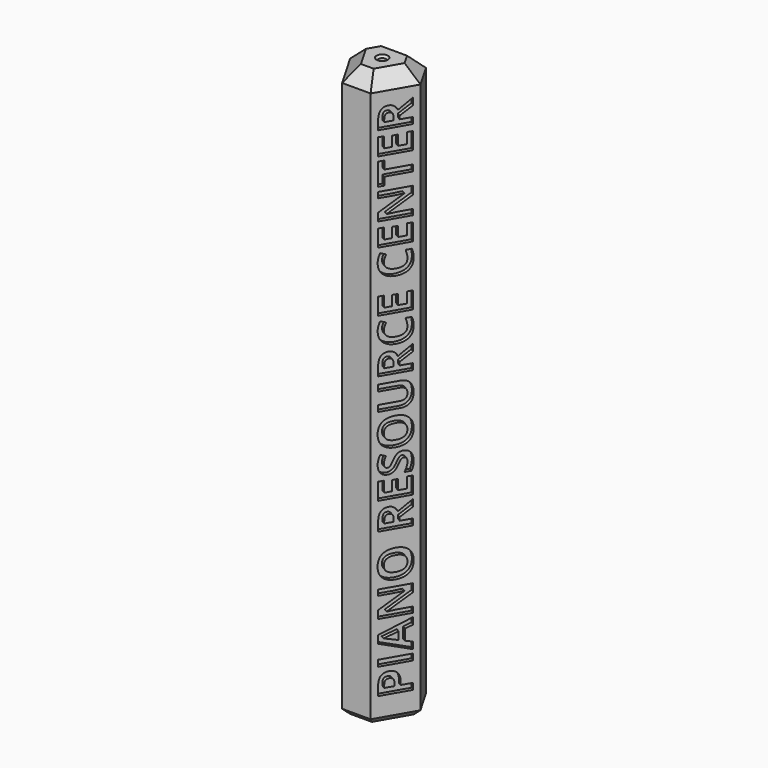
from build123d import *

# Parameters (mm, degrees)
F1_DEPTH        = 63.5
F3_D            = 4.064
F3_DEPTH        = 60.325
F3_CSINK_D      = 4.191
F3_CSINK_ANGLE  = 90
F3_TIP          = 1.2209487779
F4_SIZE         = 3.175
F5_TEXT_SIZE    = 4.5809615059
F6_DEPTH        = 0.4318
F7_TEXT_SIZE    = 4.5809615059
F8_DEPTH        = 0.4318
F9_TEXT_SIZE    = 4.5809615059
F10_DEPTH       = 0.4318
F12_D           = 0.79375
F12_CSINK_D     = 1.27
F12_CSINK_ANGLE = 90
F13_SIZE        = 0.635
F14_SIZE        = 1.524


# Not quite as in the source:
# - a feature names something its author has since deleted; it is built from what else it names
# - Text() gives the source's letters only with a copy of the font that has no kerning and outlines rounded to 1/6400 em; it was checked with that copy


with BuildPart() as f1:
    # F0 (on Top) → F1 (new body)
    with BuildSketch(Plane.XY):
        Polygon((-5.499261314, 3.175), (0, -6.35), (5.499261314, 3.175), align=None)
    extrude(amount=-F1_DEPTH)

    # F3
    with Locations(Plane(origin=(0, 0, -63.5), x_dir=(1, 0, 0), z_dir=(0, 0, -1))):
        with Locations((0, 0)):
            CounterSinkHole(F3_D / 2, F3_CSINK_D / 2, depth=F3_DEPTH, counter_sink_angle=F3_CSINK_ANGLE)
            with Locations((0, 0, -(F3_DEPTH + F3_TIP / 2))):  # 118° drill point
                Cone(0, F3_D / 2, F3_TIP, mode=Mode.SUBTRACT)

    # F4
    f4_edges = [f1.edges().sort_by_distance(p)[0] for p in [
        (0, -6.35, -31.75),
        (5.499261, 3.175, -31.75),
        (-5.499261, 3.175, -31.75),
    ]]
    chamfer(f4_edges, length=F4_SIZE)

    # F5 (on face) → F6 (cut)
    with BuildSketch(Plane(origin=(0, 3.175, 0), x_dir=(-1, 0, 0), z_dir=(0, 1, 0))):
        with Locations(Location((1.6491461421, -50.8), (0, 0, 90))):
            Text('REYBURN TOOLS', F5_TEXT_SIZE, font='Open Sans', font_style=FontStyle.BOLD, text_align=(TextAlign.LEFT, TextAlign.BOTTOM))
    extrude(amount=-F6_DEPTH, mode=Mode.SUBTRACT)

    # F7 (on face) → F8 (cut)
    with BuildSketch(Plane(origin=(-2.749630657, -1.5875, 0), x_dir=(0.5, -0.8660254038, 0), z_dir=(-0.8660254038, -0.5, 0))):
        with Locations(Location((1.6491461421, -58.2995350279), (0, 0, 90))):
            Text('REYBURN CYBERTUNER', F7_TEXT_SIZE, font='Open Sans', font_style=FontStyle.BOLD, text_align=(TextAlign.LEFT, TextAlign.BOTTOM))
    extrude(amount=-F8_DEPTH, mode=Mode.SUBTRACT)

    # F9 (on face) → F10 (cut)
    with BuildSketch(Plane(origin=(2.749630657, -1.5875, 0), x_dir=(0.5, 0.8660254038, 0), z_dir=(0.8660254038, -0.5, 0))):
        with Locations(Location((1.6491461421, -61.1415205997), (0, 0, 90))):
            Text('PIANO RESOURCE CENTER', F9_TEXT_SIZE, font='Open Sans', font_style=FontStyle.BOLD, text_align=(TextAlign.LEFT, TextAlign.BOTTOM))
    extrude(amount=-F10_DEPTH, mode=Mode.SUBTRACT)

    # F12 (through all)
    with Locations(Plane.XY):
        with Locations((0, 0)):
            CounterSinkHole(F12_D / 2, F12_CSINK_D / 2, counter_sink_angle=F12_CSINK_ANGLE)

    # F13
    f13_edges = [f1.edges().sort_by_distance(p)[0] for p in [
        (-2.749631, -1.5875, -63.5),
        (-3.118011, 1.800185, -63.5),
        (0, 3.175, -63.5),
        (3.118011, 1.800185, -63.5),
        (2.749631, -1.5875, -63.5),
        (0, -3.600369, -63.5),
    ]]
    chamfer(f13_edges, length=F13_SIZE)

    # F14
    f14_edges = [f1.edges().sort_by_distance(p)[0] for p in [
        (2.749631, -1.5875, 0),
        (0, -3.600369, 0),
        (-2.749631, -1.5875, 0),
        (-3.118011, 1.800185, 0),
        (0, 3.175, 0),
        (3.118011, 1.800185, 0),
    ]]
    chamfer(f14_edges, length=F14_SIZE)


solid = f1.part
